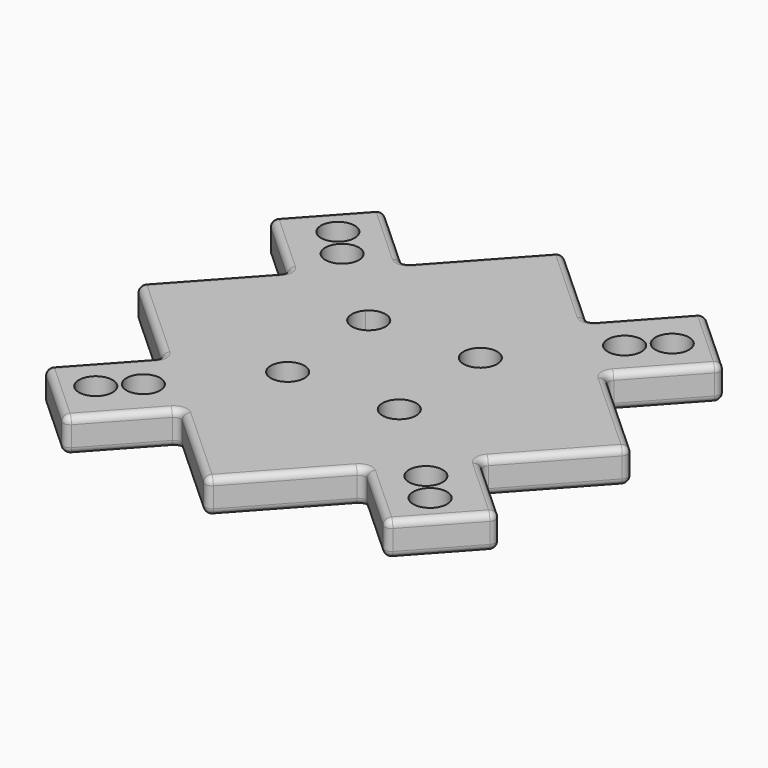
from build123d import *

# Parameters (mm, degrees)
F0_R     = 12.5
F1_DEPTH = 25
F2_F1_R  = 5
F2_F2_R  = 5


with BuildPart() as f1:
    # F0 (on Top) → F1 (new body)
    with BuildSketch(Plane.XY):
        with BuildLine():
            ThreePointArc((84.1746765519, 92.4100850957), (114.3390453191, 50.5131934796), (125, 0))
            ThreePointArc((125, 0), (116.5681360927, -45.131692278), (92.410085634, -84.1746759609))
            Line((92.410085634, -84.1746759609), (116.9144070246, -57.2729221618))
            Line((116.9144070246, -57.2729221618), (176.5847616479, 8.2354085359))
            Line((176.5847616479, 8.2354085359), (106.7917142693, 71.8086341541))
            Line((106.7917142693, 71.8086341541), (84.1746765519, 92.4100850957))
        make_face()
        with BuildLine():
            ThreePointArc((-92.410085938, 84.1746756271), (-5.8233138519, 124.864282386), (84.1746765519, 92.4100850957))
            Line((84.1746765519, 92.4100850957), (57.2729221618, 116.9144070246))
            Line((57.2729221618, 116.9144070246), (-8.2354085359, 176.5847616479))
            Line((-8.2354085359, 176.5847616479), (-71.8086341541, 106.7917142693))
            Line((-71.8086341541, 106.7917142693), (-92.410085938, 84.1746756271))
        make_face()
        Polygon((57.2729221618, 116.9144070246), (84.1746765519, 92.4100850957), (106.7917142693, 71.8086341541), (153.3977572181, 122.9744784544), (103.8789651106, 168.0802513249), align=None)
        with Locations((93.7508121133, 106.0864329338)):
            Circle(F0_R, mode=Mode.SUBTRACT)
        with Locations((113.7711524508, 125.2529812725)):
            Circle(F0_R, mode=Mode.SUBTRACT)
        with BuildLine():
            Line((71.8086341541, -106.7917142693), (92.410085634, -84.1746759609))
            ThreePointArc((92.410085634, -84.1746759609), (5.8233127337, -124.8642824382), (-84.1746778733, -92.410083892))
            Line((-84.1746778733, -92.410083892), (-57.2729221618, -116.9144070246))
            Line((-57.2729221618, -116.9144070246), (8.2354085359, -176.5847616479))
            Line((8.2354085359, -176.5847616479), (71.8086341541, -106.7917142693))
        make_face()
        Polygon((116.9144070246, -57.2729221618), (92.410085634, -84.1746759609), (71.8086341541, -106.7917142693), (122.9744784544, -153.3977572181), (168.0802513249, -103.8789651106), align=None)
        with Locations((125.2529812725, -113.7711524508)):
            Circle(F0_R, mode=Mode.SUBTRACT)
        with Locations((106.0864329338, -93.7508121133)):
            Circle(F0_R, mode=Mode.SUBTRACT)
        with BuildLine():
            ThreePointArc((-84.1746778733, -92.410083892), (-124.8642824277, -5.8233129591), (-92.410085938, 84.1746756271))
            Line((-92.410085938, 84.1746756271), (-116.9144070246, 57.2729221618))
            Line((-116.9144070246, 57.2729221618), (-176.5847616479, -8.2354085359))
            Line((-176.5847616479, -8.2354085359), (-106.7917142693, -71.8086341541))
            Line((-106.7917142693, -71.8086341541), (-84.1746778733, -92.410083892))
        make_face()
        Polygon((-116.9144070246, 57.2729221618), (-92.410085938, 84.1746756271), (-71.8086341541, 106.7917142693), (-122.9744784544, 153.3977572181), (-168.0802513249, 103.8789651106), align=None)
        with BuildLine():
            ThreePointArc((-93.5864329338, 93.7508121133), (-94.086358675, 90.2510667249), (-95.5461477792, 87.0312593857))
            ThreePointArc((-95.5461477792, 87.0312593857), (-118.0865071926, 97.2505575017), (-93.5864329338, 93.7508121133))
        make_face(mode=Mode.SUBTRACT)
        with Locations((-125.2529812725, 113.7711524508)):
            Circle(F0_R, mode=Mode.SUBTRACT)
        Polygon((-57.2729221618, -116.9144070246), (-84.1746778733, -92.410083892), (-106.7917142693, -71.8086341541), (-153.3977572181, -122.9744784544), (-103.8789651106, -168.0802513249), align=None)
        with Locations((-113.7711524508, -125.2529812725)):
            Circle(F0_R, mode=Mode.SUBTRACT)
        with Locations((-93.7508121133, -106.0864329338)):
            Circle(F0_R, mode=Mode.SUBTRACT)
        with BuildLine():
            ThreePointArc((92.410085634, -84.1746759609), (116.5681360927, -45.131692278), (125, 0))
            ThreePointArc((125, 0), (114.3390453191, 50.5131934796), (84.1746765519, 92.4100850957))
            ThreePointArc((84.1746765519, 92.4100850957), (-5.8233138519, 124.864282386), (-92.410085938, 84.1746756271))
            ThreePointArc((-92.410085938, 84.1746756271), (-124.8642824277, -5.8233129591), (-84.1746778733, -92.410083892))
            ThreePointArc((-84.1746778733, -92.410083892), (5.8233127337, -124.8642824382), (92.410085634, -84.1746759609))
        make_face()
        with BuildLine():
            ThreePointArc((-46.4980849836, -51.0473240379), (-47.3216258372, -33.3888478731), (-29.6631496724, -32.5653070196))
            ThreePointArc((-29.6631496724, -32.5653070196), (-26.646712796, -36.754996181), (-25.580617328, -41.8063155288))
            ThreePointArc((-25.580617328, -41.8063155288), (-33.0292979803, -53.2402200608), (-46.4980849836, -51.0473240379))
        make_face(mode=Mode.SUBTRACT)
        with Locations((41.8063155288, -38.080617328)):
            Circle(F0_R, mode=Mode.SUBTRACT)
        with BuildLine():
            ThreePointArc((-32.5653070196, 29.6631496724), (-50.2237831844, 28.8396088188), (-51.0473240379, 46.4980849836))
            ThreePointArc((-51.0473240379, 46.4980849836), (-37.2931462634, 49.7374309227), (-29.3063155288, 38.080617328))
            ThreePointArc((-29.3063155288, 38.080617328), (-30.149501934, 33.5674480627), (-32.5653070196, 29.6631496724))
        make_face(mode=Mode.SUBTRACT)
        with Locations((38.080617328, 41.8063155288)):
            Circle(F0_R, mode=Mode.SUBTRACT)
    extrude(amount=F1_DEPTH)

    # F2: fillet of radius 5 on 56 edges, made by hand

    # F2_f1
    f2_f1_edges = [f1.edges().sort_by_distance(p)[0] for p in [
        (-71.8086341541, 106.7917142693, 12.5),
        (57.2729221618, 116.9144070246, 12.5),
        (106.7917142693, 71.8086341541, 12.5),
        (116.9144070246, -57.2729221618, 12.5),
        (71.8086341541, -106.7917142693, 12.5),
        (-57.2729221618, -116.9144070246, 12.5),
        (-106.7917142693, -71.8086341541, 12.5),
        (-116.9144070246, 57.2729221618, 12.5),
    ]]
    fillet(f2_f1_edges, radius=F2_F1_R)

    # F2_f2
    f2_f2_edges = [f1.edges().sort_by_distance(p)[0] for p in [
        (-8.2354085359, 176.5847616479, 12.5),
        (-38.3385278139, 143.5364396605, 0),
        (-38.3385278139, 143.5364396605, 25),
        (22.6705551112, 148.4330778674, 0),
        (22.6705551112, 148.4330778674, 25),
        (103.8789651106, 168.0802513249, 12.5),
        (82.2594371674, 144.3455308766, 0),
        (82.2594371674, 144.3455308766, 25),
        (-122.9744784544, 153.3977572181, 12.5),
        (-168.0802513249, 103.8789651106, 12.5),
        (-145.5273648897, 128.6383611644, 0),
        (-145.5273648897, 128.6383611644, 25),
        (153.3977572181, 122.9744784544, 12.5),
        (128.6383611644, 145.5273648897, 0),
        (128.6383611644, 145.5273648897, 25),
        (131.7782292749, 99.2397580061, 0),
        (131.7782292749, 99.2397580061, 25),
        (176.5847616479, 8.2354085359, 12.5),
        (148.4330778674, -22.6705551112, 0),
        (148.4330778674, -22.6705551112, 25),
        (143.5364396605, 38.3385278139, 0),
        (143.5364396605, 38.3385278139, 25),
        (168.0802513249, -103.8789651106, 12.5),
        (144.3455308766, -82.2594371674, 0),
        (144.3455308766, -82.2594371674, 25),
        (122.9744784544, -153.3977572181, 12.5),
        (145.5273648897, -128.6383611644, 0),
        (145.5273648897, -128.6383611644, 25),
        (8.2354085359, -176.5847616479, 12.5),
        (38.3385278139, -143.5364396605, 0),
        (38.3385278139, -143.5364396605, 25),
        (99.2397580061, -131.7782292749, 0),
        (99.2397580061, -131.7782292749, 25),
        (-22.6705551112, -148.4330778674, 0),
        (-22.6705551112, -148.4330778674, 25),
        (-103.8789651106, -168.0802513249, 12.5),
        (-82.2594371674, -144.3455308766, 0),
        (-82.2594371674, -144.3455308766, 25),
        (-153.3977572181, -122.9744784544, 12.5),
        (-128.6383611644, -145.5273648897, 0),
        (-128.6383611644, -145.5273648897, 25),
        (-131.7782292749, -99.2397580061, 0),
        (-131.7782292749, -99.2397580061, 25),
        (-176.5847616479, -8.2354085359, 12.5),
        (-143.5364396605, -38.3385278139, 0),
        (-143.5364396605, -38.3385278139, 25),
        (-148.4330778674, 22.6705551112, 0),
        (-148.4330778674, 22.6705551112, 25),
        (-118.9832261939, 57.1764383493, 25),
        (-118.9832261939, 57.1764383493, 0),
        (-108.8605334386, -71.9051179667, 25),
        (-108.8605334386, -71.9051179667, 0),
        (-57.1764383493, -118.9832261939, 25),
        (-57.1764383493, -118.9832261939, 0),
        (71.9051179667, -108.8605334386, 25),
        (71.9051179667, -108.8605334386, 0),
        (118.9832261939, -57.1764383493, 25),
        (118.9832261939, -57.1764383493, 0),
        (108.8605334386, 71.9051179667, 25),
        (108.8605334386, 71.9051179667, 0),
        (57.1764383493, 118.9832261939, 25),
        (57.1764383493, 118.9832261939, 0),
        (-71.9051179667, 108.8605334386, 25),
        (-71.9051179667, 108.8605334386, 0),
    ]]
    fillet(f2_f2_edges, radius=F2_F2_R)


solid = f1.part
